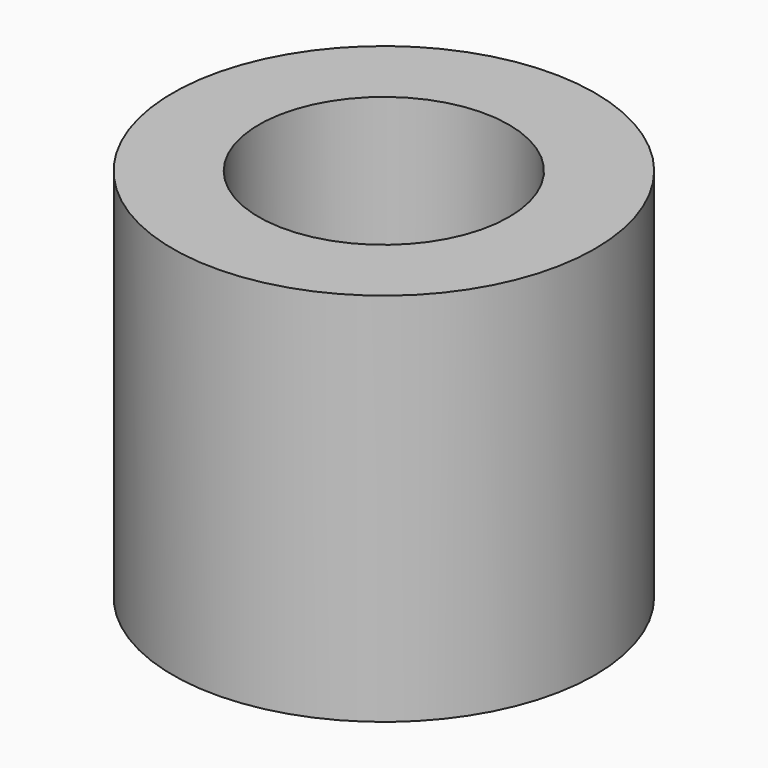
from build123d import *

# Parameters (mm, degrees)
F1_R     = 10.715625
F1_R_2   = 6.35
F2_DEPTH = 19.05


# Not quite as in the source:
# - a variable given as a bare number and used for a length is read in inches; the dataset says mm whatever the document's units were


with BuildPart() as f2:
    # F1 (on Top) → F2 (new body)
    with BuildSketch(Plane.XY):
        Circle(F1_R)
        Circle(F1_R_2, mode=Mode.SUBTRACT)
    extrude(amount=F2_DEPTH)


solid = f2.part
